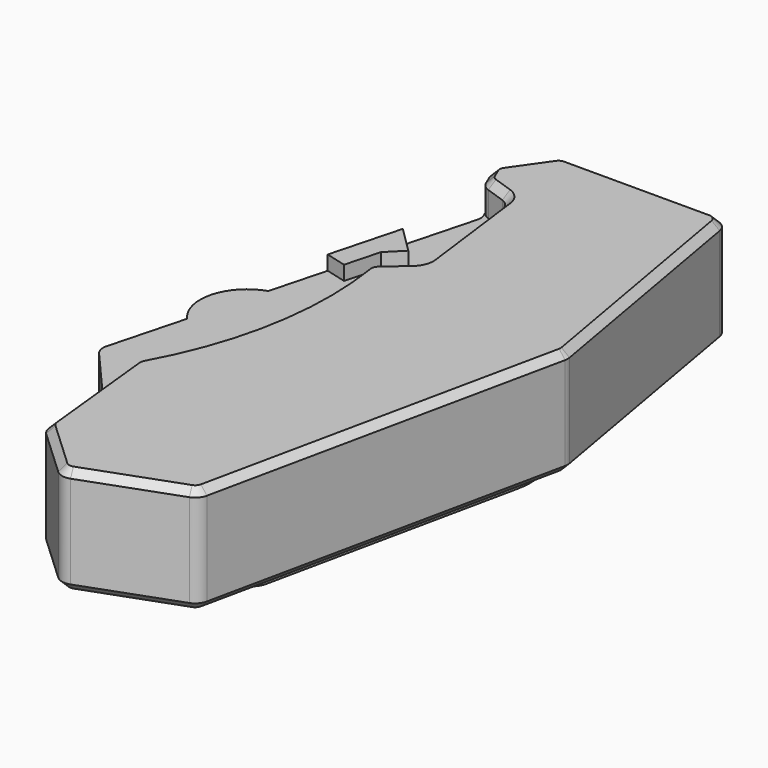
from build123d import *

# Parameters (mm, degrees)
F1_DEPTH       = 15
F2_R           = 2
F4_DEPTH       = 4.5
F6_DEPTH       = 4.5
F7_R           = 2
F8_SIZE        = 1
F10_DEPTH      = 2
F10_DEPTH_BACK = 8
F12_DEPTH      = 5
F14_DEPTH      = 1
F15_R          = 10
F16_R          = 3
F17_R          = 2
F18_T1_DEPTH   = 27


# Not quite as in the source:
# - a fillet or chamfer that OpenCascade refuses, or shapes differently, is made with other operations: its cross-section is extruded or revolved along the edge and cut away or added


with BuildPart() as f1:
    # F0 (on Top) → F1 (new body)
    with BuildSketch(Plane.XY):
        Polygon((-8.0448907178, 7.5019819607), (0, 0), (15.0350819326, 5.4723222932), (25.8464898551, 56.3359975314), (19.5579639798, 92), (-3.4420360202, 92), (-8.030647511, 85.4467836457), (-6.4537553867, 81.7707244475), (-13.8947211419, 53.7415962301), (-16.7171564284, 43.1098579407), (-19.7961767409, 31.5115979887), (-9.299232277, 19.4362447051), align=None)
        with BuildLine():
            ThreePointArc((-13.8947211419, 53.7415962301), (-18.2055037731, 49.1954821635), (-16.7171564284, 43.1098579407))
            Line((-16.7171564284, 43.1098579407), (-13.8947211419, 53.7415962301))
        make_face()
    extrude(amount=F1_DEPTH)

    # F2
    f2_edges = [f1.edges().sort_by_distance(p)[0] for p in [
        (-3.442036, 92, 7.5),
        (19.557964, 92, 7.5),
        (-8.030648, 85.446784, 7.5),
        (-6.453755, 81.770724, 7.5),
        (25.84649, 56.335998, 7.5),
        (15.035082, 5.472322, 7.5),
        (-19.796177, 31.511598, 7.5),
        (-8.044891, 7.501982, 7.5),
        (0, 0, 7.5),
    ]]
    fillet(f2_edges, radius=F2_R)

    # F3 (on face) → F4 (cut)
    with BuildSketch(Plane.XY.offset(15)):
        with BuildLine():
            Line((-19.1004557272, 30.7112625143), (-9.299232277, 19.4362447051))
            Line((-9.299232277, 19.4362447051), (-9.9431083431, 25.5623162612))
            ThreePointArc((-9.9431083431, 25.5623162612), (-4.1654007718, 41.7730592838), (-4.2262892289, 58.9825446545))
            Line((-4.2262892289, 58.9825446545), (0.2837840411, 62.9397203012))
            Line((0.2837840411, 62.9397203012), (-1.9921549357, 80.795254507))
            Line((-1.9921549357, 80.795254507), (-6.7258938789, 82.4051351292))
            ThreePointArc((-6.7258938789, 82.4051351292), (-6.5692308005, 81.7622951194), (-6.6308801526, 81.103519015))
            Line((-6.6308801526, 81.103519015), (-13.8947211419, 53.7415962301))
            ThreePointArc((-13.8947211419, 53.7415962301), (-18.2055037731, 49.1954821635), (-16.7171564284, 43.1098579407))
            Line((-16.7171564284, 43.1098579407), (-19.5240798921, 32.5365506243))
            ThreePointArc((-19.5240798921, 32.5365506243), (-19.539255282, 31.5712259114), (-19.1004557272, 30.7112625143))
        make_face()
    extrude(amount=-F4_DEPTH, mode=Mode.SUBTRACT)

    # F5 (on face) → F6 (cut)
    with BuildSketch(Plane(origin=(0, 0, 0), x_dir=(1, 0, 0), z_dir=(0, 0, -1))):
        with BuildLine():
            ThreePointArc((-6.6308801526, -81.103519015), (-6.5692308005, -81.7622951194), (-6.7258938789, -82.4051351292))
            Line((-6.7258938789, -82.4051351292), (-2.0079532375, -80.7495276563))
            Line((-2.0079532375, -80.7495276563), (0.2709017201, -62.8943653752))
            Line((0.2709017201, -62.8943653752), (-4.2385252382, -58.9364532352))
            ThreePointArc((-4.2385252382, -58.9364532352), (-4.1797341848, -41.7514896804), (-9.9430388376, -25.5616549609))
            Line((-9.9430388376, -25.5616549609), (-9.299232277, -19.4362447051))
            Line((-9.299232277, -19.4362447051), (-19.1004557272, -30.7112625143))
            ThreePointArc((-19.1004557272, -30.7112625143), (-19.539255282, -31.5712259114), (-19.5240798921, -32.5365506243))
            Line((-19.5240798921, -32.5365506243), (-16.7171564284, -43.1098579407))
            ThreePointArc((-16.7171564284, -43.1098579407), (-18.2055037731, -49.1954821635), (-13.8947211419, -53.7415962301))
            Line((-13.8947211419, -53.7415962301), (-6.6308801526, -81.103519015))
        make_face()
    extrude(amount=-F6_DEPTH, mode=Mode.SUBTRACT)

    # F7
    f7_edges = [f1.edges().sort_by_distance(p)[0] for p in [
        (-9.943108, 25.562316, 12.75),
        (-9.943039, 25.561655, 2.25),
        (-4.226289, 58.982545, 12.75),
        (0.283784, 62.93972, 12.75),
        (-4.238525, 58.936453, 2.25),
        (0.270902, 62.894365, 2.25),
        (-1.992155, 80.795255, 12.75),
        (-2.007953, 80.749528, 2.25),
        (-6.725894, 82.405135, 7.5),
        (-6.725894, 82.405135, 2.25),
        (-6.725894, 82.405135, 12.75),
    ]]
    fillet(f7_edges, radius=F7_R)

    # F8
    f8_edges = [f1.edges().sort_by_distance(p)[0] for p in [
        (-7.334289, 83.82343, 15),
        (-6.597337, 82.544049, 15),
        (-7.743054, 85.417108, 15),
        (-4.528565, 81.657853, 15),
        (-5.715563, 88.753067, 15),
        (-2.269238, 80.568943, 15),
        (-3.324399, 91.774022, 15),
        (-0.842477, 71.775634, 15),
        (7.739431, 92, 15),
        (0.035819, 63.033597, 15),
        (19.16534, 91.532089, 15),
        (-1.952405, 60.977669, 15),
        (22.814181, 73.533074, 15),
        (-3.950317, 58.895605, 15),
        (25.809062, 56.336651, 15),
        (-4.205609, 41.541288, 15),
        (20.515619, 31.256223, 15),
        (-9.848308, 25.536603, 15),
        (14.818701, 5.66042, 15),
        (-8.999956, 16.588822, 15),
        (7.572505, 2.756166, 15),
        (-7.923879, 7.562316, 15),
        (0.068913, 0.338716, 15),
        (-4.197178, 3.913931, 15),
        (-7.332009, 83.818114, 0),
        (-6.599862, 82.540006, 0),
        (-7.743054, 85.417108, 0),
        (-4.534925, 81.636286, 0),
        (-5.715563, 88.753067, 0),
        (-2.280519, 80.529059, 0),
        (-3.324399, 91.774022, 0),
        (-0.857666, 71.736857, 0),
        (7.739431, 92, 0),
        (0.022922, 62.988201, 0),
        (19.16534, 91.532089, 0),
        (-1.965224, 60.931724, 0),
        (22.814181, 73.533074, 0),
        (-3.962878, 58.849592, 0),
        (25.809062, 56.336651, 0),
        (-4.219912, 41.519712, 0),
        (20.515619, 31.256223, 0),
        (-9.848432, 25.536019, 0),
        (14.818701, 5.66042, 0),
        (-8.999957, 16.588832, 0),
        (7.572505, 2.756166, 0),
        (-7.923879, 7.562316, 0),
        (0.068913, 0.338716, 0),
        (-4.197178, 3.913931, 0),
    ]]
    chamfer(f8_edges, length=F8_SIZE)

    # F9 (on face) → F10 (join, two sides)
    with BuildSketch(Plane.XY.offset(10.5)) as f10_sk:
        Polygon((-9.2121738851, 71.3801288833), (-11.82835392, 61.5253266909), (-8.928788932, 60.7555716127), (-7.6458638018, 65.5881799261), (-5.5294538555, 67.7143993266), align=None)
    extrude(amount=F10_DEPTH)
    extrude(f10_sk.sketch, amount=-F10_DEPTH_BACK)

    # F11 (on face) → F12 (join)
    with BuildSketch(Plane(origin=(0, 0, 0), x_dir=(1, 0, 0), z_dir=(0, 0, -1))):
        Polygon((5.5166269788, -69.1855618273), (14.7091602962, -76.8990131435), (15.3519479059, -76.1329687004), (6.1594145885, -68.4195173842), align=None)
    extrude(amount=F12_DEPTH)

    # F13 (on face) → F14 (join)
    with BuildSketch(Plane(origin=(0, 0, -5), x_dir=(1, 0, 0), z_dir=(0, 0, -1))):
        Polygon((6.1594145885, -68.4195173842), (15.3519479059, -76.1329687004), (18.3099562872, -59.3572695449), (9.9443103961, -20), (4.371628125, -21.1845101828), (8.5288556293, -61.3816455007), align=None)
        Polygon((14.7091602962, -76.8990131435), (15.3519479059, -76.1329687004), (6.1594145885, -68.4195173842), (5.5166269788, -69.1855618273), align=None)
    extrude(amount=-F14_DEPTH)

    # F15
    f15_edges = [f1.edges().sort_by_distance(p)[0] for p in [
        (18.309956, 59.35727, -4.5),
        (8.528856, 61.381646, -4.5),
    ]]
    fillet(f15_edges, radius=F15_R)

    # F16
    f16_edges = [f1.edges().sort_by_distance(p)[0] for p in [
        (4.371628, 21.18451, -4.5),
        (9.94431, 20, -4.5),
    ]]
    fillet(f16_edges, radius=F16_R)

    # F17
    f17_edges = [f1.edges().sort_by_distance(p)[0] for p in [
        (10.755681, 72.276243, -4),
    ]]
    fillet(f17_edges, radius=F17_R)

    # F18: fillet of radius 3 on 1 edges, made by hand

    # F18_s2 → F18_t1 (cut)
    with BuildSketch(Plane(origin=(31.5591951189, 26.4813089845, 0), x_dir=(0, 0, 1), z_dir=(0.7660444431, 0.6427876097, 0))):
        with BuildLine():
            ThreePointArc((-5, -46.4531957126), (-4.1213203436, -48.5745160562), (-2, -49.4531957126))
            Line((-2, -49.4531957126), (-5, -49.4531957126))
            Line((-5, -49.4531957126), (-5, -46.4531957126))
        make_face()
    extrude(amount=F18_T1_DEPTH, mode=Mode.SUBTRACT)


solid = f1.part
